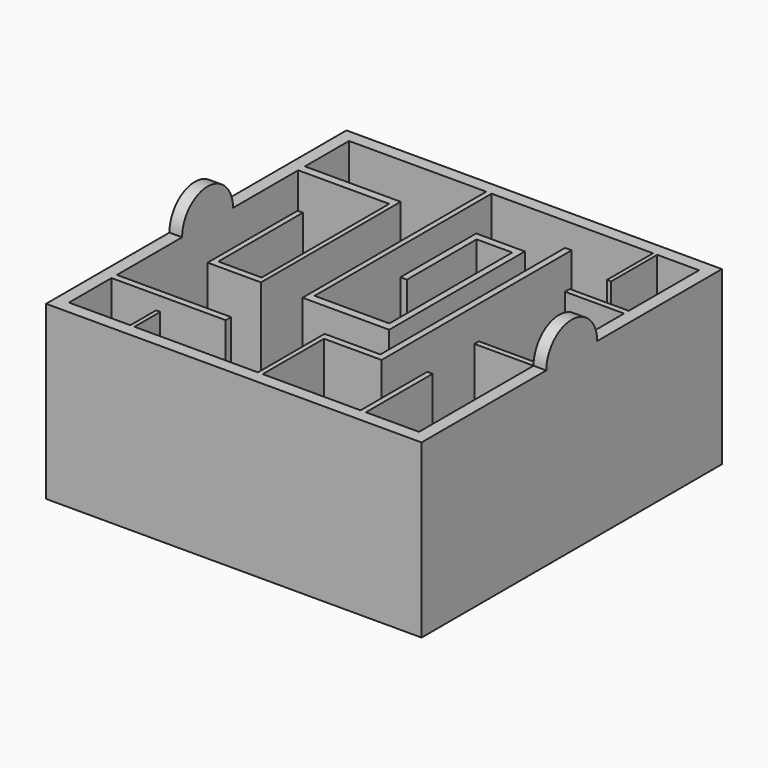
from build123d import *

# Parameters (mm, degrees)
F0_W      = 55
F0_H      = 55
F1_DEPTH  = 2
F2_W      = 0.8393637836
F2_H      = 13.1056420505
F2_W_2    = 14.2980124801
F2_H_2    = 1.318924129
F2_W_3    = 17.9352443665
F2_H_3    = 1.0551437736
F2_W_4    = 0.6528366357
F2_H_4    = 5.0601772964
F2_W_5    = 1.0258853436
F2_H_5    = 24.1364017129
F2_W_6    = 0.7460992783
F2_H_6    = 12.0504982769
F2_W_7    = 8.0205630511
F2_W_8    = 9.2725682259
F2_H_7    = 0.9232535958
F2_W_9    = 0.6528384984
F2_H_8    = 9.0530256927
F2_W_10   = 9.2923234403
F2_H_9    = 0.8714348078
F3_DEPTH  = 25
F5_DEPTH  = 2
F7_DEPTH  = 25
F8_W      = 57
F8_H      = 2
F9_DEPTH  = 2
F10_W     = 2
F10_H     = 57
F11_DEPTH = 25
F13_DEPTH = 2
F15_DEPTH = 25
F17_DEPTH = 2
F19_DEPTH = 25
F20_W     = 5.9659110848
F20_H     = 4.5738629997
F21_DEPTH = 25
F24_DEPTH = 2
F26_DEPTH = 2


with BuildPart() as f1:
    # F0 (on Top) → F1 (new body)
    with BuildSketch(Plane.XY):
        with Locations((27.5, 27.5)):
            Rectangle(F0_W, F0_H)
    extrude(amount=F1_DEPTH)

    # F2 (on face) → F3 (join)
    with BuildSketch(Plane.XY.offset(2)):
        with Locations((46.2403725833, 6.5528210253)):
            Rectangle(F2_W, F2_H)
        with Locations((7.1490062401, 45.6831902266)):
            Rectangle(F2_W_2, F2_H_2)
        Polygon((15.0441108271, 46.3426522911), (14.2980124801, 46.3426522911), (14.2980124801, 45.0237281621), (14.2980124801, 19.9640728533), (15.0441108271, 19.9640728533), align=None)
        Polygon((15.0441108271, 19.9640728533), (14.2980124801, 19.9640728533), (7.4898591265, 19.9640728533), (7.4898591265, 18.9089290798), (15.0441108271, 18.9089290798), align=None)
        Polygon((7.4898591265, 18.9089290798), (7.4898591265, 19.9640728533), (7.4898591265, 36.5825779736), (6.6504976712, 36.5825779736), (6.6504976712, 18.9089290798), align=None)
        with Locations((8.9676221833, 8.8850706816)):
            Rectangle(F2_W_3, F2_H_3)
        with Locations((9.9613117054, 2.5300886482)):
            Rectangle(F2_W_4, F2_H_4)
        Polygon((22.4118363112, 55), (21.5724762529, 55), (21.5724762529, 18.9089290798), (22.4118363112, 18.9089290798), (22.4118363112, 20.2278606594), align=None)
        Polygon((34.1628938913, 20.2278606594), (22.4118363112, 20.2278606594), (22.4118363112, 18.9089290798), (35.1887792349, 18.9089290798), (35.1887792349, 20.2278606594), align=None)
        with Locations((34.6758365631, 32.2960615158)):
            Rectangle(F2_W_5, F2_H_5)
        Polygon((28.5671520978, 44.3642623723), (34.1628938913, 44.3642623723), (35.1887792349, 44.3642623723), (35.1887792349, 45.5512963235), (28.5671520978, 45.5512963235), align=None)
        Polygon((28.5671520978, 30.6474007666), (28.5671520978, 44.3642623723), (28.5671520978, 45.5512963235), (27.5412686169, 45.5512963235), (27.5412686169, 30.6474007666), align=None)
        with Locations((30.0593515858, 6.0252491385)):
            Rectangle(F2_W_6, F2_H_6)
        with Locations((30.0593515858, 12.5780701637)):
            Rectangle(F2_W_6, F2_H_3)
        with Locations((34.4426827505, 12.5780701637)):
            Rectangle(F2_W_7, F2_H_3)
        Polygon((38.4529642761, 13.1056420505), (38.4529642761, 12.0504982769), (39.4788496196, 12.0504982769), (39.4788496196, 49.376193434), (38.4529642761, 49.376193434), align=None)
        with Locations((50.3637158871, 40.7372042537)):
            Rectangle(F2_W_8, F2_H_7)
        with Locations((48.1056179851, 50.4734871536)):
            Rectangle(F2_W_9, F2_H_8)
        with Locations((50.3538382798, 22.9402892292)):
            Rectangle(F2_W_10, F2_H_9)
    extrude(amount=F3_DEPTH)

    # F4 (on face) → F5 (join)
    with BuildSketch(Plane.XZ):
        Polygon((9.6348933876, 2), (0, 2), (0, 0), (55, 0), (55, 2), (46.6600544751, 2), (45.8206906915, 2), (30.432401225, 2), (29.6863019466, 2), (10.2877300233, 2), align=None)
    extrude(amount=F5_DEPTH)

    # F6 (on face) → F7 (join)
    with BuildSketch(Plane.XY.offset(2)):
        Polygon((9.6348933876, 0), (0, 0), (0, -2), (55, -2), (55, 0), (46.6600544751, 0), (45.8206906915, 0), (30.432401225, 0), (29.6863019466, 0), (10.2877300233, 0), align=None)
    extrude(amount=F7_DEPTH)

    # F8 (on face) → F9 (join)
    with BuildSketch(Plane(origin=(0, 0, 0), x_dir=(0, -1, 0), z_dir=(-1, 0, 0))):
        with Locations((-26.5, 1)):
            Rectangle(F8_W, F8_H)
    extrude(amount=F9_DEPTH)

    # F10 (on face) → F11 (join)
    with BuildSketch(Plane.XY.offset(2)):
        with Locations((-1, 26.5)):
            Rectangle(F10_W, F10_H)
    extrude(amount=F11_DEPTH)

    # F12 (on face) → F13 (join)
    with BuildSketch(Plane(origin=(0, 55, 0), x_dir=(-1, 0, 0), z_dir=(0, 1, 0))):
        Polygon((-55, 0), (2, 0), (2, 2), (0, 2), (-21.5724762529, 2), (-22.4118363112, 2), (-47.779198736, 2), (-48.4320372343, 2), (-55, 2), align=None)
    extrude(amount=F13_DEPTH)

    # F14 (on face) → F15 (join)
    with BuildSketch(Plane.XY.offset(2)):
        Polygon((55, 55), (55, 57), (-2, 57), (-2, 55), (0, 55), (21.5724762529, 55), (22.4118363112, 55), (47.779198736, 55), (48.4320372343, 55), align=None)
    extrude(amount=F15_DEPTH)

    # F16 (on face) → F17 (join)
    with BuildSketch(Plane.YZ.offset(55)):
        Polygon((-2, 2), (-2, 0), (57, 0), (57, 2), (55, 2), (41.1988310516, 2), (40.2755774558, 2), (23.376006633, 2), (22.5045718253, 2), (0, 2), align=None)
    extrude(amount=F17_DEPTH)

    # F18 (on face) → F19 (join)
    with BuildSketch(Plane.XY.offset(2)):
        Polygon((57, -2), (57, 57), (55, 57), (55, 55), (55, 41.1988310516), (55, 40.2755774558), (55, 23.376006633), (55, 22.5045718253), (55, 0), (55, -2), align=None)
    extrude(amount=F19_DEPTH)

    # F20 (on face) → F21 (cut)
    with BuildSketch(Plane.XY.offset(2)):
        with Locations((6.1647732509, 50.411934033)):
            Rectangle(F20_W, F20_H)
    extrude(amount=-F21_DEPTH, mode=Mode.SUBTRACT)

    # F23 (on face) → F24 (join, through all)
    with BuildSketch(Plane.YZ.offset(57)):
        with BuildLine():
            Line((22.5, 27), (32.5, 27))
            ThreePointArc((32.5, 27), (27.5, 32), (22.5, 27))
        make_face()
        with BuildLine():
            Line((57, 27), (32.5, 27))
            ThreePointArc((32.5, 27), (27.5, 22), (22.5, 27))
            Line((22.5, 27), (-2, 27))
            Line((-2, 27), (-2, 0))
            Line((-2, 0), (57, 0))
            Line((57, 0), (57, 27))
        make_face()
    extrude(amount=-F24_DEPTH)

    # F25 (on face) → F26 (join, through all)
    with BuildSketch(Plane.YZ):
        with BuildLine():
            Line((22.2181853652, 27), (32.2181853652, 27))
            ThreePointArc((32.2181853652, 27), (27.2181853652, 32), (22.2181853652, 27))
        make_face()
    extrude(amount=-F26_DEPTH)


solid = f1.part
